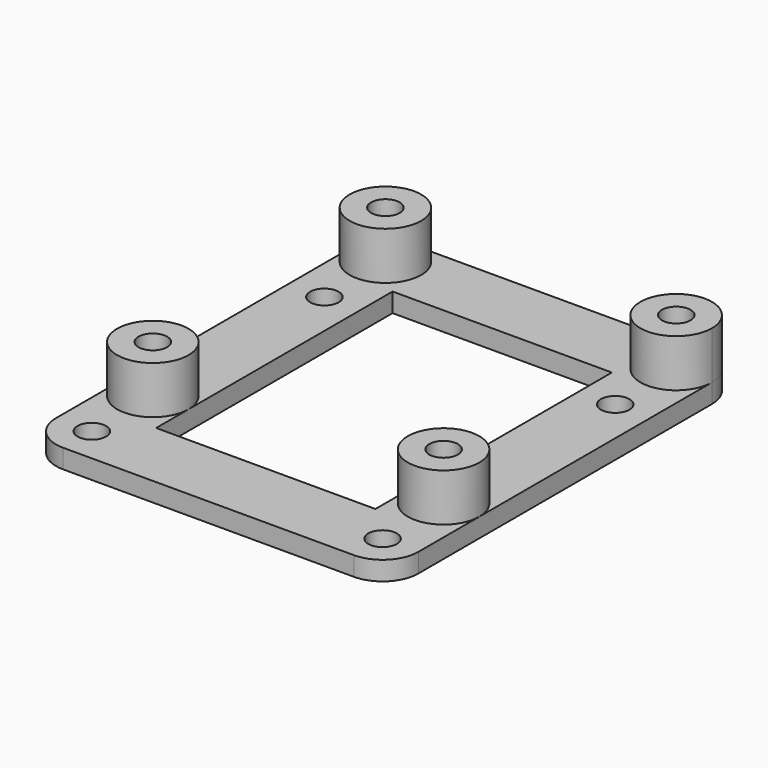
from build123d import *

# Parameters (mm, degrees)
F3_W     = 38
F3_H     = 46
F3_R     = 1.5
F3_W_2   = 23
F3_H_2   = 31
F4_DEPTH = 2
F5_R     = 1.5
F6_DEPTH = 5
F7_R     = 3.7499
F8_R     = 3.1
F9_DEPTH = 5


# Not quite as in the source:
# - a fillet or chamfer is up to 0.001 mm smaller than in the source, because OpenCascade refuses the exact size


with BuildPart() as f4:
    # F3 (on Top) → F4 (new body)
    with BuildSketch(Plane.XY):
        Rectangle(F3_W, F3_H)
        with Locations((-15.25, -19.25)):
            Circle(F3_R, mode=Mode.SUBTRACT)
        with Locations((-15.25, -11.25)):
            Circle(F3_R, mode=Mode.SUBTRACT)
        with Locations((15.25, -19.25)):
            Circle(F3_R, mode=Mode.SUBTRACT)
        with Locations((15.25, -11.25)):
            Circle(F3_R, mode=Mode.SUBTRACT)
        with Locations((-15.25, 11.25)):
            Circle(F3_R, mode=Mode.SUBTRACT)
        with Locations((-15.25, 19.25)):
            Circle(F3_R, mode=Mode.SUBTRACT)
        Rectangle(F3_W_2, F3_H_2, mode=Mode.SUBTRACT)
        with Locations((15.25, 11.25)):
            Circle(F3_R, mode=Mode.SUBTRACT)
        with Locations((15.25, 19.25)):
            Circle(F3_R, mode=Mode.SUBTRACT)
    extrude(amount=F4_DEPTH)

    # F5 (on face) → F6 (join)
    with BuildSketch(Plane.XY.offset(2)):
        with BuildLine():
            ThreePointArc((-19, 19.25), (-15.25, 15.5), (-11.5, 19.25))
            ThreePointArc((-11.5, 19.25), (-12.598349559, 21.9016504179), (-15.2499999673, 23))
            ThreePointArc((-15.2499999673, 23), (-17.9016504179, 21.901650441), (-19, 19.25))
        make_face()
        with Locations((-15.25, 19.25)):
            Circle(F5_R, mode=Mode.SUBTRACT)
        with BuildLine():
            ThreePointArc((19, 19.25), (17.9016504294, 21.9016504294), (15.25, 23))
            ThreePointArc((15.25, 23), (12.5983495706, 16.5983495706), (19, 19.25))
        make_face()
        with Locations((15.25, 19.25)):
            Circle(F5_R, mode=Mode.SUBTRACT)
        with BuildLine():
            ThreePointArc((11.5, -11.25), (15.25, -15), (19, -11.25))
            ThreePointArc((19, -11.25), (15.25, -7.5), (11.5, -11.25))
        make_face()
        with Locations((15.25, -11.25)):
            Circle(F5_R, mode=Mode.SUBTRACT)
        with BuildLine():
            ThreePointArc((-11.5, -11.25), (-15.2499999923, -7.5), (-19, -11.2499999846))
            ThreePointArc((-19, -11.2499999846), (-15.2500000077, -15), (-11.5, -11.25))
        make_face()
        with Locations((-15.25, -11.25)):
            Circle(F5_R, mode=Mode.SUBTRACT)
    extrude(amount=F6_DEPTH)

    # F7 (radius 3.75 in the source; OpenCascade refuses exactly that, so slightly less here)
    f7_edges = [f4.edges().sort_by_distance(p)[0] for p in [
        (-19, 23, 1),
        (-19, -23, 1),
        (19, -23, 1),
        (19, 23, 1),
    ]]
    fillet(f7_edges, radius=F7_R)

    # F8 (on face) → F9 (cut)
    with BuildSketch(Plane(origin=(0, 0, 0), x_dir=(1, 0, 0), z_dir=(0, 0, -1))):
        with Locations((-15.25, 11.25)):
            Circle(F8_R)
        with Locations((15.25, 11.25)):
            Circle(F8_R)
        with Locations((15.25, -19.25)):
            Circle(F8_R)
        with Locations((-15.25, -19.25)):
            Circle(F8_R)
    extrude(amount=-F9_DEPTH, mode=Mode.SUBTRACT)


solid = f4.part
